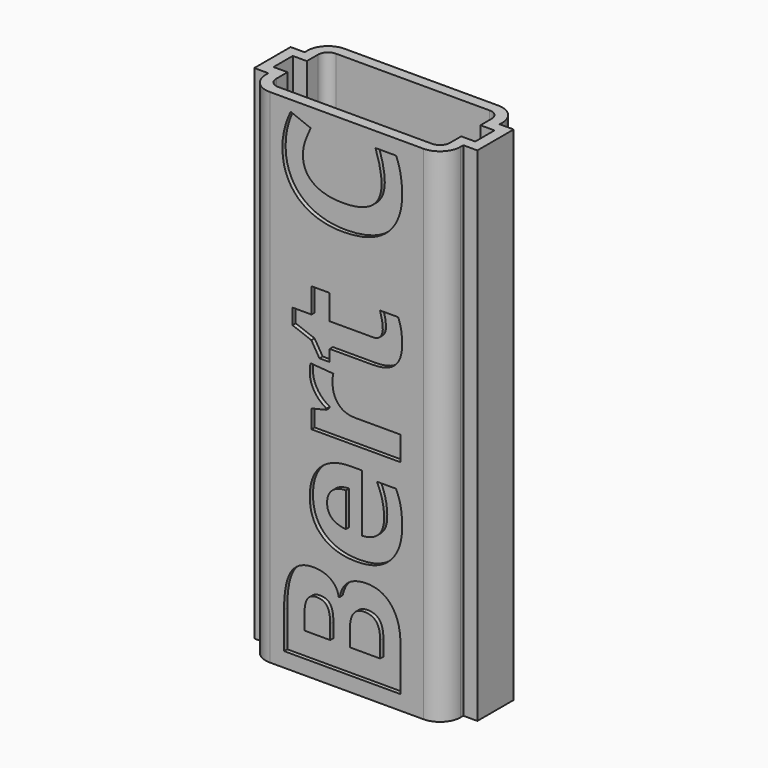
from build123d import *

# Parameters (mm, degrees)
F1_DEPTH     = 36.6
F0_W         = 0.55
F0_H         = 0.4
F2_DEPTH     = 1
F3_TEXT_SIZE = 12.2177091795
F4_DEPTH     = 0.3


# Not quite as in the source:
# - Text() gives the source's letters only with a copy of the font that has no kerning and outlines rounded to 1/6400 em; it was checked with that copy


with BuildPart() as f1:
    # F0 (on Top) → F1 (new body)
    with BuildSketch(Plane.XY):
        with BuildLine():
            Line((-3.5608965084, 11.1282052323), (-15.0608965084, 11.1282052323))
            ThreePointArc((-15.0608965084, 11.1282052323), (-16.1569120192, 10.6742207432), (-16.6108965084, 9.5782052323))
            Line((-16.6108965084, 9.5782052323), (-16.6108965084, 9.3282052323))
            Line((-16.6108965084, 9.3282052323), (-17.6608965084, 9.3282052323))
            Line((-17.6608965084, 9.3282052323), (-17.6608965084, 7.6282052323))
            Line((-17.6608965084, 7.6282052323), (-17.6608965084, 5.9282052323))
            Line((-17.6608965084, 5.9282052323), (-16.6108965084, 5.9282052323))
            Line((-16.6108965084, 5.9282052323), (-16.6108965084, 5.6782052323))
            ThreePointArc((-16.6108965084, 5.6782052323), (-16.1569120192, 4.5821897215), (-15.0608965084, 4.1282052323))
            Line((-15.0608965084, 4.1282052323), (-3.5608965084, 4.1282052323))
            ThreePointArc((-3.5608965084, 4.1282052323), (-2.4648809976, 4.5821897215), (-2.0108965084, 5.6782052323))
            Line((-2.0108965084, 5.6782052323), (-2.0108965084, 5.9282052323))
            Line((-2.0108965084, 5.9282052323), (-0.9608965084, 5.9282052323))
            Line((-0.9608965084, 5.9282052323), (-0.9608965084, 7.6282052323))
            Line((-0.9608965084, 7.6282052323), (-0.9608965084, 9.3282052323))
            Line((-0.9608965084, 9.3282052323), (-2.0108965084, 9.3282052323))
            Line((-2.0108965084, 9.3282052323), (-2.0108965084, 9.5782052323))
            ThreePointArc((-2.0108965084, 9.5782052323), (-2.4648809976, 10.6742207432), (-3.5608965084, 11.1282052323))
        make_face()
        with BuildLine():
            Line((-16.8608965084, 8.5282052323), (-15.8108965084, 8.5282052323))
            Line((-15.8108965084, 8.5282052323), (-15.8108965084, 9.5782052323))
            ThreePointArc((-15.8108965084, 9.5782052323), (-15.5912265943, 10.1085353182), (-15.0608965084, 10.3282052323))
            Line((-15.0608965084, 10.3282052323), (-3.5608965084, 10.3282052323))
            ThreePointArc((-3.5608965084, 10.3282052323), (-3.0305664225, 10.1085353182), (-2.8108965084, 9.5782052323))
            Line((-2.8108965084, 9.5782052323), (-2.8108965084, 8.5282052323))
            Line((-2.8108965084, 8.5282052323), (-1.7608965084, 8.5282052323))
            Line((-1.7608965084, 8.5282052323), (-1.7608965084, 7.6282052323))
            Line((-1.7608965084, 7.6282052323), (-1.7608965084, 6.7282052323))
            Line((-1.7608965084, 6.7282052323), (-2.8108965084, 6.7282052323))
            Line((-2.8108965084, 6.7282052323), (-2.8108965084, 5.6782052323))
            ThreePointArc((-2.8108965084, 5.6782052323), (-3.0305664225, 5.1478751464), (-3.5608965084, 4.9282052323))
            Line((-3.5608965084, 4.9282052323), (-15.0608965084, 4.9282052323))
            ThreePointArc((-15.0608965084, 4.9282052323), (-15.5912265943, 5.1478751464), (-15.8108965084, 5.6782052323))
            Line((-15.8108965084, 5.6782052323), (-15.8108965084, 6.7282052323))
            Line((-15.8108965084, 6.7282052323), (-16.8608965084, 6.7282052323))
            Line((-16.8608965084, 6.7282052323), (-16.8608965084, 7.6282052323))
            Line((-16.8608965084, 7.6282052323), (-16.8608965084, 8.5282052323))
        make_face(mode=Mode.SUBTRACT)
    extrude(amount=F1_DEPTH)

    # F0 (on Top) → F2 (join)
    with BuildSketch(Plane.XY):
        with BuildLine():
            Line((-3.5608965084, 11.1282052323), (-15.0608965084, 11.1282052323))
            ThreePointArc((-15.0608965084, 11.1282052323), (-16.1569120192, 10.6742207432), (-16.6108965084, 9.5782052323))
            Line((-16.6108965084, 9.5782052323), (-16.6108965084, 9.3282052323))
            Line((-16.6108965084, 9.3282052323), (-17.6608965084, 9.3282052323))
            Line((-17.6608965084, 9.3282052323), (-17.6608965084, 7.6282052323))
            Line((-17.6608965084, 7.6282052323), (-17.6608965084, 5.9282052323))
            Line((-17.6608965084, 5.9282052323), (-16.6108965084, 5.9282052323))
            Line((-16.6108965084, 5.9282052323), (-16.6108965084, 5.6782052323))
            ThreePointArc((-16.6108965084, 5.6782052323), (-16.1569120192, 4.5821897215), (-15.0608965084, 4.1282052323))
            Line((-15.0608965084, 4.1282052323), (-3.5608965084, 4.1282052323))
            ThreePointArc((-3.5608965084, 4.1282052323), (-2.4648809976, 4.5821897215), (-2.0108965084, 5.6782052323))
            Line((-2.0108965084, 5.6782052323), (-2.0108965084, 5.9282052323))
            Line((-2.0108965084, 5.9282052323), (-0.9608965084, 5.9282052323))
            Line((-0.9608965084, 5.9282052323), (-0.9608965084, 7.6282052323))
            Line((-0.9608965084, 7.6282052323), (-0.9608965084, 9.3282052323))
            Line((-0.9608965084, 9.3282052323), (-2.0108965084, 9.3282052323))
            Line((-2.0108965084, 9.3282052323), (-2.0108965084, 9.5782052323))
            ThreePointArc((-2.0108965084, 9.5782052323), (-2.4648809976, 10.6742207432), (-3.5608965084, 11.1282052323))
        make_face()
        with BuildLine():
            Line((-16.8608965084, 8.5282052323), (-15.8108965084, 8.5282052323))
            Line((-15.8108965084, 8.5282052323), (-15.8108965084, 9.5782052323))
            ThreePointArc((-15.8108965084, 9.5782052323), (-15.5912265943, 10.1085353182), (-15.0608965084, 10.3282052323))
            Line((-15.0608965084, 10.3282052323), (-3.5608965084, 10.3282052323))
            ThreePointArc((-3.5608965084, 10.3282052323), (-3.0305664225, 10.1085353182), (-2.8108965084, 9.5782052323))
            Line((-2.8108965084, 9.5782052323), (-2.8108965084, 8.5282052323))
            Line((-2.8108965084, 8.5282052323), (-1.7608965084, 8.5282052323))
            Line((-1.7608965084, 8.5282052323), (-1.7608965084, 7.6282052323))
            Line((-1.7608965084, 7.6282052323), (-1.7608965084, 6.7282052323))
            Line((-1.7608965084, 6.7282052323), (-2.8108965084, 6.7282052323))
            Line((-2.8108965084, 6.7282052323), (-2.8108965084, 5.6782052323))
            ThreePointArc((-2.8108965084, 5.6782052323), (-3.0305664225, 5.1478751464), (-3.5608965084, 4.9282052323))
            Line((-3.5608965084, 4.9282052323), (-15.0608965084, 4.9282052323))
            ThreePointArc((-15.0608965084, 4.9282052323), (-15.5912265943, 5.1478751464), (-15.8108965084, 5.6782052323))
            Line((-15.8108965084, 5.6782052323), (-15.8108965084, 6.7282052323))
            Line((-15.8108965084, 6.7282052323), (-16.8608965084, 6.7282052323))
            Line((-16.8608965084, 6.7282052323), (-16.8608965084, 7.6282052323))
            Line((-16.8608965084, 7.6282052323), (-16.8608965084, 8.5282052323))
        make_face(mode=Mode.SUBTRACT)
        Polygon((-16.3608965084, 8.0282052323), (-15.8108965084, 8.0282052323), (-15.8108965084, 8.5282052323), (-16.8608965084, 8.5282052323), (-16.8608965084, 7.6282052323), (-16.8608965084, 6.7282052323), (-15.8108965084, 6.7282052323), (-15.8108965084, 7.2282052323), (-16.3608965084, 7.2282052323), (-16.3608965084, 7.6282052323), align=None)
        with Locations((-16.0858965084, 7.8282052323)):
            Rectangle(F0_W, F0_H)
        with Locations((-16.0858965084, 7.4282052323)):
            Rectangle(F0_W, F0_H)
        with Locations((-2.5358965084, 7.8282052323)):
            Rectangle(F0_W, F0_H)
        with Locations((-2.5358965084, 7.4282052323)):
            Rectangle(F0_W, F0_H)
        Polygon((-2.8108965084, 8.5282052323), (-2.8108965084, 8.0282052323), (-2.2608965084, 8.0282052323), (-2.2608965084, 7.6282052323), (-2.2608965084, 7.2282052323), (-2.8108965084, 7.2282052323), (-2.8108965084, 6.7282052323), (-1.7608965084, 6.7282052323), (-1.7608965084, 7.6282052323), (-1.7608965084, 8.5282052323), align=None)
    extrude(amount=-F2_DEPTH)

    # F3 (on face) → F4 (cut)
    with BuildSketch(Plane.XZ.offset(-4.1282052323)):
        with Locations(Location((-5.2706459309, -1), (0, 0, 90))):
            Text('Bert C', F3_TEXT_SIZE, font='Open Sans', font_style=FontStyle.BOLD, text_align=(TextAlign.LEFT, TextAlign.BOTTOM))
    extrude(amount=-F4_DEPTH, mode=Mode.SUBTRACT)


solid = f1.part
